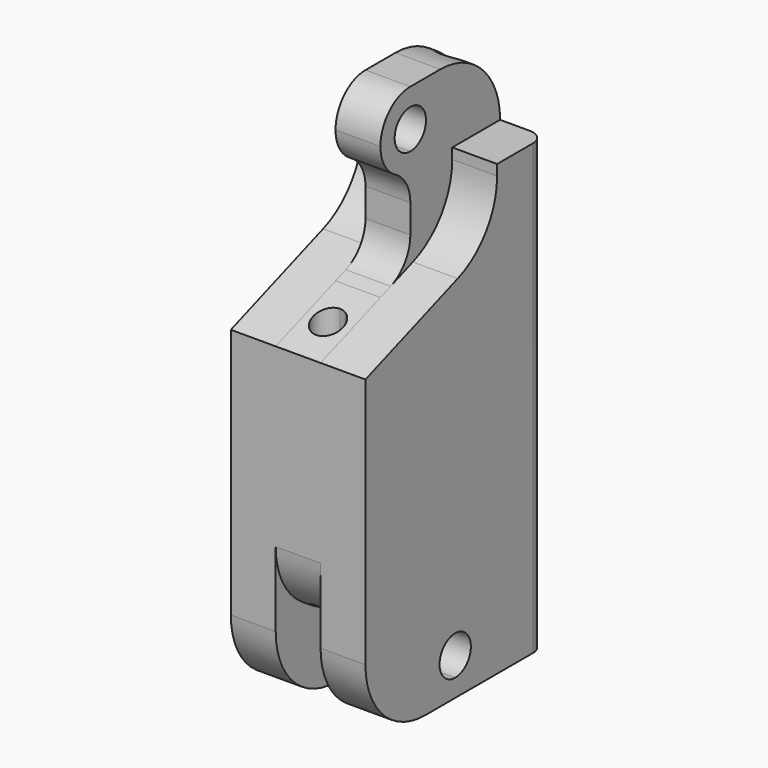
from build123d import *

# Parameters (mm, degrees)
F1_DEPTH     = 15
F3_DEPTH     = 6
F5_DEPTH     = 18
F6_R         = 10
F9_DEPTH     = 6
F10_DEPTH    = 6
F11_R        = 2
F13_DEPTH    = 6
F15_R        = 10
F19_DEPTH    = 65.001
F21_DEPTH    = 60.001
F23_DEPTH    = 6
F24_T1_DEPTH = 6


# Not quite as in the source:
# - a fillet or chamfer that OpenCascade refuses, or shapes differently, is made with other operations: its cross-section is extruded or revolved along the edge and cut away or added


with BuildPart() as f1:
    # F0 (on Front) → F1 (new body, symmetric)
    with BuildSketch(Plane.XZ):
        Polygon((9, -25), (9, 25), (3, 25), (3, 35), (-3, 35), (-3, 25), (-9, 25), (-9, -25), (-9, -35), (-3, -35), (-3, -25), (3, -25), (3, -35), (9, -35), align=None)
    extrude(amount=F1_DEPTH, both=True)

    # F2 (on face) → F3 (cut)
    with BuildSketch(Plane(origin=(-3, 0, 0), x_dir=(0, -1, 0), z_dir=(-1, 0, 0))):
        with BuildLine():
            ThreePointArc((0, 32.62), (-2.62, 30), (0, 27.38))
            Line((0, 27.38), (0, 32.62))
        make_face()
        with BuildLine():
            Line((0, 32.62), (0, 27.38))
            ThreePointArc((0, 27.38), (1.8526197667, 28.1473802333), (2.62, 30))
            ThreePointArc((2.62, 30), (1.8526197667, 31.8526197667), (0, 32.62))
        make_face()
    extrude(amount=-F3_DEPTH, mode=Mode.SUBTRACT)

    # F4 (on face) → F5 (cut)
    with BuildSketch(Plane(origin=(-9, 0, 0), x_dir=(0, -1, 0), z_dir=(-1, 0, 0))):
        with BuildLine():
            ThreePointArc((0, -32.62), (1.8526197667, -31.8526197667), (2.62, -30))
            ThreePointArc((2.62, -30), (-1.8526197667, -28.1473802333), (0, -32.62))
        make_face()
    extrude(amount=-F5_DEPTH, mode=Mode.SUBTRACT)

    # F6
    f6_edges = [f1.edges().sort_by_distance(p)[0] for p in [
        (0, 15, 35),
        (0, -15, 35),
        (6, -15, -35),
        (-6, -15, -35),
    ]]
    fillet(f6_edges, radius=F6_R)

    # F8 (on face) → F9 (cut)
    with BuildSketch(Plane(origin=(-9, 0, 0), x_dir=(0, -1, 0), z_dir=(-1, 0, 0))):
        with BuildLine():
            ThreePointArc((-7, 23.5872004348), (-5.1915204429, 17.8514360713), (-0.4202014333, 14.190274227))
            Line((-0.4202014333, 14.190274227), (15, 8.5777798989))
            Line((15, 8.5777798989), (15, 25))
            Line((15, 25), (-7, 25))
            Line((-7, 25), (-7, 23.5872004348))
        make_face()
    extrude(amount=-F9_DEPTH, mode=Mode.SUBTRACT)

    # F7 (on face) → F10 (cut)
    with BuildSketch(Plane.YZ.offset(9)):
        with BuildLine():
            Line((7, 25), (-15, 25))
            Line((-15, 25), (-15, 8.57778))
            Line((-15, 8.57778), (0.4202014333, 14.1902743281))
            ThreePointArc((0.4202014333, 14.1902743281), (5.1915204429, 17.8514361724), (7, 23.587200536))
            Line((7, 23.587200536), (7, 25))
        make_face()
    extrude(amount=-F10_DEPTH, mode=Mode.SUBTRACT)

    # F11
    f11_edges = [f1.edges().sort_by_distance(p)[0] for p in [
        (9, 15, -5),
        (-9, 15, -5),
    ]]
    fillet(f11_edges, radius=F11_R)

    # F12 (on face) → F13 (cut)
    with BuildSketch(Plane(origin=(-3, 0, 0), x_dir=(0, -1, 0), z_dir=(-1, 0, 0))):
        with BuildLine():
            Line((5, 35), (0, 35))
            ThreePointArc((0, 35), (3.5355339059, 33.5355339059), (5, 30))
            Line((5, 30), (5, 12.2174822415))
            Line((5, 12.2174822415), (15, 8.5777798989))
            Line((15, 8.5777798989), (15, 25))
            ThreePointArc((15, 25), (12.0710678119, 32.0710678119), (5, 35))
        make_face()
    extrude(amount=-F13_DEPTH, mode=Mode.SUBTRACT)

    # F15
    f15_edges = [f1.edges().sort_by_distance(p)[0] for p in [
        (0, -15, -25),
    ]]
    fillet(f15_edges, radius=F15_R)

    # F18 (on face) → F19 (cut, through all)
    with BuildSketch(Plane.XY.offset(30)):
        with BuildLine():
            ThreePointArc((2, -10), (1.4142135624, -8.5857864376), (0, -8))
            Line((0, -8), (0, -12))
            ThreePointArc((0, -12), (1.4142135624, -11.4142135624), (2, -10))
        make_face()
        with BuildLine():
            Line((0, -12), (0, -8))
            ThreePointArc((0, -8), (-2, -10), (0, -12))
        make_face()
    extrude(amount=-F19_DEPTH, mode=Mode.SUBTRACT)

    # F20 (on face) → F21 (cut, through all)
    with BuildSketch(Plane(origin=(0, 0, -25), x_dir=(1, 0, 0), z_dir=(0, 0, -1))):
        with BuildLine():
            ThreePointArc((0, -9), (-2, -11), (0, -13))
            Line((0, -13), (0, -11))
            Line((0, -11), (0, -9))
        make_face()
        with BuildLine():
            Line((0, -11), (0, -13))
            ThreePointArc((0, -13), (1.4142135624, -12.4142135624), (2, -11))
            ThreePointArc((2, -11), (1.4142135624, -9.5857864376), (0, -9))
            Line((0, -9), (0, -11))
        make_face()
    extrude(amount=-F21_DEPTH, mode=Mode.SUBTRACT)

    # F22 (on face) → F23 (cut)
    with BuildSketch(Plane.YZ.offset(3)):
        with BuildLine():
            ThreePointArc((0, 25), (-3.5355339059, 26.4644660941), (-5, 30))
            Line((-5, 30), (-5, 12.2174822415))
            Line((-5.0000000325, 12.2174823308), (0, 14.037333514))
            Line((0, 14.037333514), (0, 25))
        make_face()
    extrude(amount=-F23_DEPTH, mode=Mode.SUBTRACT)

    # F24: fillet of radius 5 on 2 edges, made by hand

    # F24_s2 → F24_t1 (join)
    with BuildSketch(Plane.YZ.offset(-3)):
        with BuildLine():
            ThreePointArc((-2.5, 25.6698729811), (-0.6698729811, 23.8397459622), (0, 21.3397459622))
            Line((0, 21.3397459622), (0, 25))
            ThreePointArc((0, 25), (-1.2940952255, 25.1703708686), (-2.5, 25.6698729811))
        make_face()
        with BuildLine():
            ThreePointArc((-3.2898992834, 12.8399081011), (-0.9042397786, 14.6704890233), (0, 17.538371205))
            Line((0, 17.538371205), (0, 14.037333514))
            Line((0, 14.037333514), (-3.2898992834, 12.8399081011))
        make_face()
    extrude(amount=F24_T1_DEPTH)


solid = f1.part
